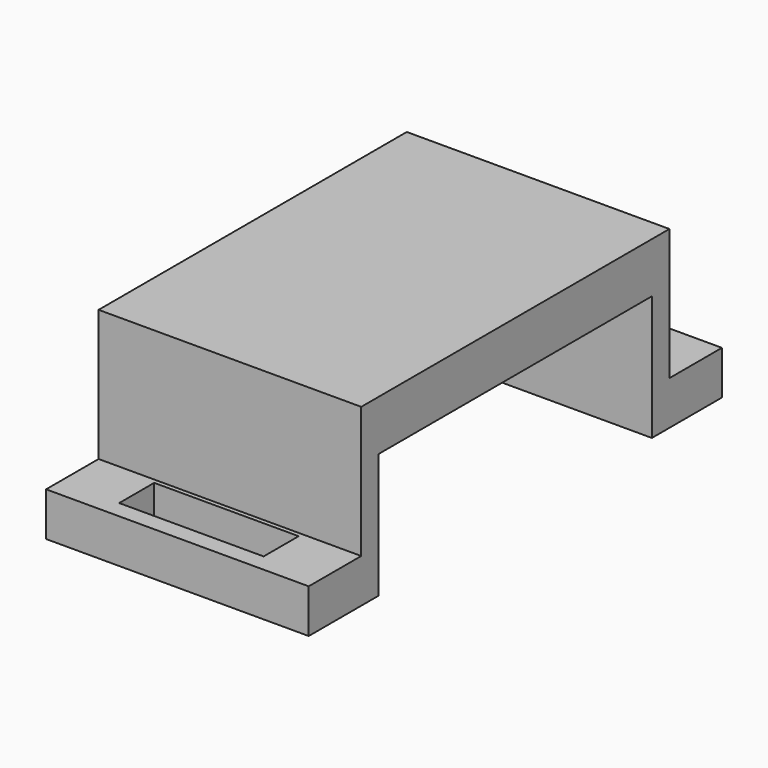
from build123d import *

# Parameters (mm, degrees)
F0_W      = 60
F0_H      = 88
F1_DEPTH  = 40
F2_W      = 80.694272792
F2_H      = 78
F3_DEPTH  = 28.5
F5_W      = 60
F5_H      = 10
F6_DEPTH  = 15
F8_W      = 60
F8_H      = 10
F9_DEPTH  = 15
F10_W     = 31
F10_H     = 10
F11_DEPTH = 25


# Not quite as in the source:
# - a pattern or mirror of a feature is missing from the dataset's text; its kind, count and spacing are read off the source's solid


with BuildPart() as f1:
    # F0 (on Top) → F1 (new body)
    with BuildSketch(Plane.XY):
        Rectangle(F0_W, F0_H)
    extrude(amount=F1_DEPTH)

    # F2 (on Top) → F3 (cut)
    with BuildSketch(Plane.XY):
        with Locations((-10.347136396, 0)):
            Rectangle(F2_W, F2_H)
    extrude(amount=F3_DEPTH, mode=Mode.SUBTRACT)

    # F5 (on offset) → F6 (join)
    with BuildSketch(Plane.XZ.offset(44)):
        with Locations((0, 5)):
            Rectangle(F5_W, F5_H)
    extrude(amount=F6_DEPTH)

    # F8 (on offset) → F9 (join)
    with BuildSketch(Plane.XZ.offset(-44)):
        with Locations((0, 5)):
            Rectangle(F8_W, F8_H)
    extrude(amount=-F9_DEPTH)

    # F10 (on Top) → F11 (cut)
    with BuildSketch(Plane.XY):
        with Locations((-1, -50)):
            Rectangle(F10_W, F10_H)
        with Locations((-1, 50)):
            Rectangle(F10_W, F10_H)
    f11 = extrude(amount=F11_DEPTH, mode=Mode.SUBTRACT)

    # F11_copies: F11 across plane
    add(f11.mirror(Plane(origin=(0, 0, 0), x_dir=(0, 0, 1), z_dir=(1, 0, 0))), mode=Mode.SUBTRACT)


solid = f1.part
